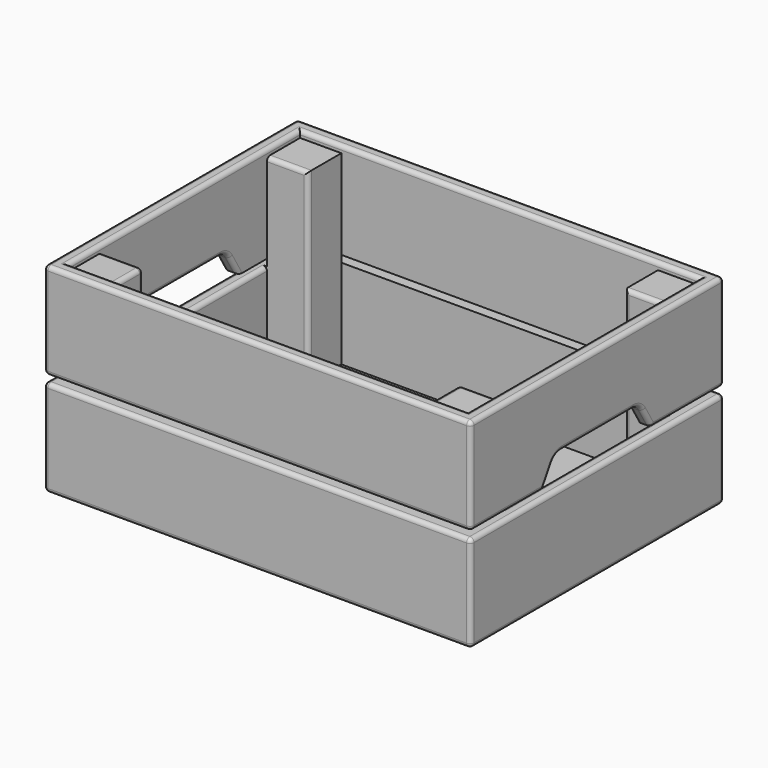
from build123d import *

# Parameters (mm, degrees)
F0_W      = 310
F0_H      = 230
F2_DEPTH  = 145
F1_W      = 290
F1_H      = 210
F3_DEPTH  = 5
F4_W      = 289.9999934435
F4_H      = 209.9999934435
F5_DEPTH  = 140
F7_DEPTH  = 310.001
F9_START  = 15
F8_W      = 30
F8_H      = 30
F9_DEPTH  = 120
F10_W     = 30
F10_H     = 209.9999934435
F11_DEPTH = 15
F12_R     = 3


with BuildPart() as f2:
    # F0 (on Top) → F2 (new body)
    with BuildSketch(Plane.XY):
        Rectangle(F0_W, F0_H)
    extrude(amount=F2_DEPTH)

    # F1 (on face) → F3 (join)
    with BuildSketch(Plane.XY):
        Rectangle(F1_W, F1_H)
    extrude(amount=-F3_DEPTH)

    # F4 (on face) → F5 (cut)
    with BuildSketch(Plane.XY.offset(145)):
        Rectangle(F4_W, F4_H)
    extrude(amount=-F5_DEPTH, mode=Mode.SUBTRACT)

    # F6 (on face) → F7 (cut, through all)
    with BuildSketch(Plane.YZ.offset(155)):
        with BuildLine():
            Line((-49, 75), (-115, 75))
            Line((-115, 75), (-115, 70))
            Line((-115, 70), (115, 70))
            Line((115, 70), (115, 75))
            Line((115, 75), (49, 75))
            Line((49, 75), (40.9071192856, 88.6107539288))
            ThreePointArc((40.9071192856, 88.6107539288), (37.256073336, 92.1921671431), (32.3117604054, 93.5))
            Line((32.3117604054, 93.5), (-32.3117604054, 93.5))
            ThreePointArc((-32.3117604054, 93.5), (-37.256073336, 92.1921671431), (-40.9071192856, 88.6107539288))
            Line((-40.9071192856, 88.6107539288), (-49, 75))
        make_face()
    extrude(amount=-F7_DEPTH, mode=Mode.SUBTRACT)

    # F8 (on face) → F9 (join)
    with BuildSketch(Plane.XY.offset(5).offset(F9_START)):
        with Locations((-129.9999967217, 89.9999967217)):
            Rectangle(F8_W, F8_H)
        with Locations((129.9999967217, 89.9999967217)):
            Rectangle(F8_W, F8_H)
        with Locations((129.9999967217, -89.9999967217)):
            Rectangle(F8_W, F8_H)
        with Locations((-129.9999967217, -89.9999967217)):
            Rectangle(F8_W, F8_H)
    extrude(amount=F9_DEPTH)

    # F10 (on face) → F11 (join)
    with BuildSketch(Plane.XY.offset(5)):
        Polygon((114.9999967217, -74.9999967217), (114.9999967217, -104.9999967217), (144.9999967217, -104.9999967217), (144.9999967217, 104.9999967217), (114.9999967217, 104.9999967217), align=None)
        with Locations((-129.9999967217, 0)):
            Rectangle(F10_W, F10_H)
    extrude(amount=F11_DEPTH)

    # F12
    f12_edges = [f2.edges().sort_by_distance(p)[0] for p in [
        (155, 0, 0),
        (155, 115, 35),
        (155, 0, 70),
        (155, -115, 35),
        (155, -82, 75),
        (155, -44.95356, 81.805377),
        (155, -37.256073, 92.192167),
        (155, 0, 93.5),
        (155, 37.256073, 92.192167),
        (155, 44.95356, 81.805377),
        (155, 82, 75),
        (155, 115, 110),
        (155, 0, 145),
        (155, -115, 110),
        (0, -115, 0),
        (0, -115, 70),
        (-155, -115, 35),
        (0, -115, 75),
        (0, -115, 145),
        (-155, -115, 110),
        (-155, 82, 75),
        (-155, 44.95356, 81.805377),
        (-155, 37.256073, 92.192167),
        (-155, 0, 93.5),
        (-155, -37.256073, 92.192167),
        (-155, -44.95356, 81.805377),
        (-155, -82, 75),
        (-155, 0, 145),
        (-155, 115, 110),
        (-155, 0, 0),
        (-155, 0, 70),
        (-155, 115, 35),
        (0, 115, 0),
        (0, 115, 70),
        (0, 115, 75),
        (0, 115, 145),
        (0, 104.999997, 145),
        (144.999997, 0, 145),
        (0, -104.999997, 145),
        (-144.999997, 0, 145),
        (-129.999997, -74.999997, 140),
        (-114.999997, -89.999997, 140),
        (-114.999997, -74.999997, 80),
        (114.999997, -89.999997, 140),
        (114.999997, -74.999997, 80),
        (129.999997, -74.999997, 140),
        (114.999997, 0, 20),
        (114.999997, 74.999997, 80),
        (129.999997, 74.999997, 140),
        (-114.999997, 0, 20),
        (-114.999997, 74.999997, 80),
        (-129.999997, 74.999997, 140),
        (144.999997, 0, 70),
        (-144.999997, 0, 70),
        (-144.999997, 37.256073, 92.192167),
        (144.999997, 37.256073, 92.192167),
        (149.999998, -49, 75),
        (149.999998, 49, 75),
        (0, 105, -5),
        (-145, 0, -5),
        (0, -105, -5),
        (145, 0, -5),
        (-149.999998, -49, 75),
        (-149.999998, 49, 75),
        (144.999997, 44.95356, 81.805377),
        (144.999997, 0, 93.5),
        (144.999997, -37.256073, 92.192167),
        (144.999997, -44.95356, 81.805377),
        (-144.999997, -44.95356, 81.805377),
        (-144.999997, -37.256073, 92.192167),
        (-144.999997, 0, 93.5),
        (-144.999997, 44.95356, 81.805377),
    ]]
    fillet(f12_edges, radius=F12_R)


solid = f2.part
